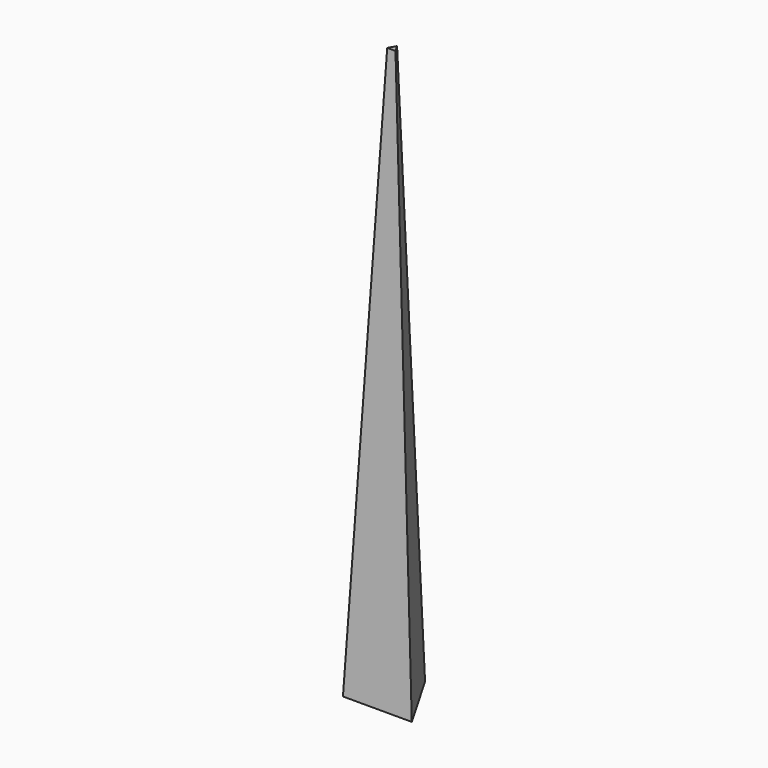
from build123d import *

# Parameters (mm, degrees)
F1_DEPTH = 250
F2_SIZE2 = 249.99999
F2_SIZE  = 7.61999
F3_SIZE2 = 249.99999
F3_SIZE  = 7.61999
F4_SIZE2 = 249.99999
F4_SIZE  = 7.61999


# Not quite as in the source:
# - a fillet or chamfer is up to 0.001 mm smaller than in the source, because OpenCascade refuses the exact size


with BuildPart() as f1:
    # F0 (on Top) → F1 (new body)
    with BuildSketch(Plane.XY):
        Polygon((-28.8751734727, 18.8044057646), (-43.8751734727, 44.7851678781), (-58.8751734727, 18.8044057646), align=None)
    extrude(amount=F1_DEPTH)

    # F2 (size 7.62 and 250 in the source; OpenCascade refuses exactly that, so slightly less here)
    f2_edges = [f1.edges().sort_by_distance(p)[0] for p in [
        (-51.375173, 31.794787, 250),
    ]]
    f2_side = f1.faces().sort_by_distance((-43.875173, 27.46466, 250))[0]
    chamfer(f2_edges, length=F2_SIZE, length2=F2_SIZE2, reference=f2_side)

    # F3 (size 7.62 and 250 in the source; OpenCascade refuses exactly that, so slightly less here)
    f3_edges = [f1.edges().sort_by_distance(p)[0] for p in [
        (-34.175472, 27.984792, 250),
    ]]
    f3_side = f1.faces().sort_by_distance((-39.47577, 24.924663, 250))[0]
    chamfer(f3_edges, length=F3_SIZE, length2=F3_SIZE2, reference=f3_side)

    # F4 (size 7.62 and 250 in the source; OpenCascade refuses exactly that, so slightly less here)
    f4_edges = [f1.edges().sort_by_distance(p)[0] for p in [
        (-43.875173, 18.804406, 250),
    ]]
    f4_side = f1.faces().sort_by_distance((-43.875173, 22.384666, 250))[0]
    chamfer(f4_edges, length=F4_SIZE, length2=F4_SIZE2, reference=f4_side)


solid = f1.part
